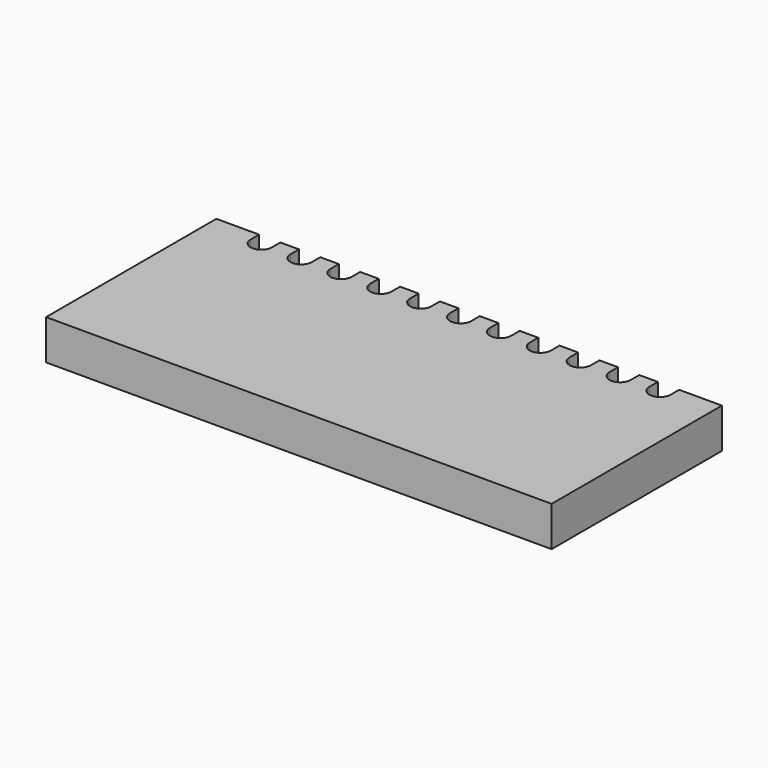
from build123d import *

# Parameters (mm, degrees)
F1_DEPTH = 1.5


with BuildPart() as f1:
    # F0 (on Top) → F1 (new body)
    with BuildSketch(Plane.XY):
        with BuildLine():
            Line((-7.893, 4), (-9.5, 4))
            Line((-9.5, 4), (-9.5, -4))
            Line((-9.5, -4), (9.5, -4))
            Line((9.5, -4), (9.5, 4))
            Line((9.5, 4), (7.893, 4))
            Line((7.893, 4), (7.893, 3.6))
            ThreePointArc((7.893, 3.6), (7.493, 3.2), (7.093, 3.6))
            Line((7.093, 3.6), (7.093, 4))
            Line((7.093, 4), (6.3944, 4))
            Line((6.3944, 4), (6.3944, 3.6))
            ThreePointArc((6.3944, 3.6), (5.9944, 3.2), (5.5944, 3.6))
            Line((5.5944, 3.6), (5.5944, 4))
            Line((5.5944, 4), (4.8958, 4))
            Line((4.8958, 4), (4.8958, 3.6))
            ThreePointArc((4.8958, 3.6), (4.4958, 3.2), (4.0958, 3.6))
            Line((4.0958, 3.6), (4.0958, 4))
            Line((4.0958, 4), (3.3972, 4))
            Line((3.3972, 4), (3.3972, 3.6))
            ThreePointArc((3.3972, 3.6), (2.9972, 3.2), (2.5972, 3.6))
            Line((2.5972, 3.6), (2.5972, 4))
            Line((2.5972, 4), (1.8986, 4))
            Line((1.8986, 4), (1.8986, 3.6))
            ThreePointArc((1.8986, 3.6), (1.4986, 3.2), (1.0986, 3.6))
            Line((1.0986, 3.6), (1.0986, 4))
            Line((1.0986, 4), (0.4, 4))
            Line((0.4, 4), (0.4, 3.6))
            ThreePointArc((0.4, 3.6), (0, 3.2), (-0.4, 3.6))
            Line((-0.4, 3.6), (-0.4, 4))
            Line((-0.4, 4), (-1.0986, 4))
            Line((-1.0986, 4), (-1.0986, 3.6))
            ThreePointArc((-1.0986, 3.6), (-1.4986, 3.2), (-1.8986, 3.6))
            Line((-1.8986, 3.6), (-1.8986, 4))
            Line((-1.8986, 4), (-2.5972, 4))
            Line((-2.5972, 4), (-2.5972, 3.6))
            ThreePointArc((-2.5972, 3.6), (-2.9972, 3.2), (-3.3972, 3.6))
            Line((-3.3972, 3.6), (-3.3972, 4))
            Line((-3.3972, 4), (-4.0958, 4))
            Line((-4.0958, 4), (-4.0958, 3.6))
            ThreePointArc((-4.0958, 3.6), (-4.4958, 3.2), (-4.8958, 3.6))
            Line((-4.8958, 3.6), (-4.8958, 4))
            Line((-4.8958, 4), (-5.5944, 4))
            Line((-5.5944, 4), (-5.5944, 3.6))
            ThreePointArc((-5.5944, 3.6), (-5.9944, 3.2), (-6.3944, 3.6))
            Line((-6.3944, 3.6), (-6.3944, 4))
            Line((-6.3944, 4), (-7.093, 4))
            Line((-7.093, 4), (-7.093, 3.6))
            ThreePointArc((-7.093, 3.6), (-7.493, 3.2), (-7.893, 3.6))
            Line((-7.893, 3.6), (-7.893, 4))
        make_face()
    extrude(amount=F1_DEPTH)


solid = f1.part
